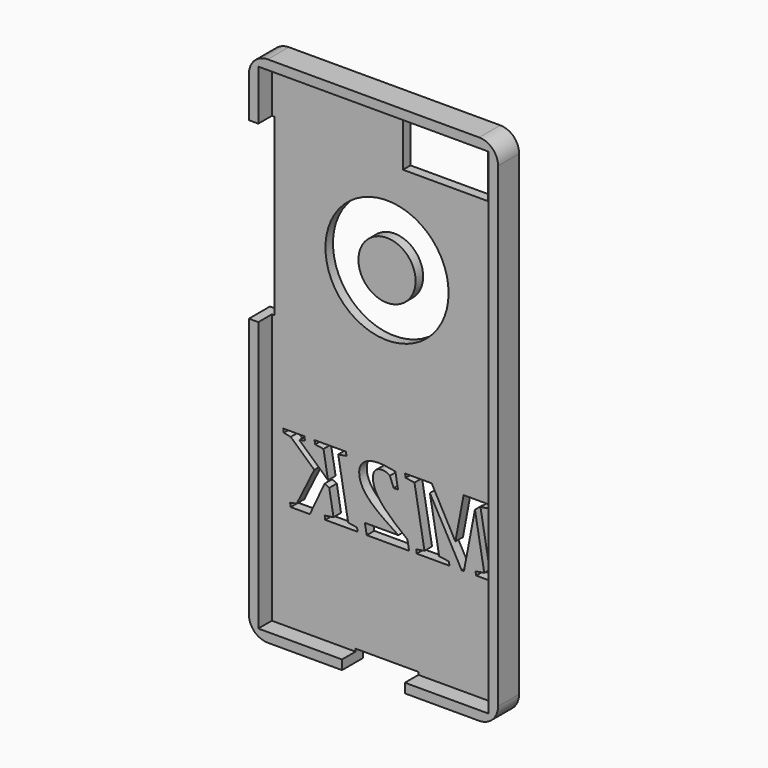
from build123d import *

# Parameters (mm, degrees)
F0_W          = 67.1
F0_H          = 138.3
F1_DEPTH      = 3.55
F2_T          = -2.54
F3_R          = 5.08
F4_W          = 22.9508173652
F4_H          = 12.0491795242
F5_DEPTH      = 12.5
F6_W          = 16.9322472066
F6_H          = 7.1
F7_DEPTH      = 3.25
F8_W          = 7.1
F8_H          = 47.0491815358
F9_DEPTH      = 3.25
F10_R         = 16.5823645395
F10_R_2       = 7.6979390502
F11_DEPTH     = 12.5
F12_TEXT_SIZE = 27.4609729899
F13_DEPTH     = 12.5


# Not quite as in the source:
# - Text() gives the source's letters only with a copy of the font that has no kerning and outlines rounded to 1/6400 em; it was checked with that copy


with BuildPart() as f1:
    # F0 (on Front) → F1 (new body, symmetric)
    with BuildSketch(Plane.XZ):
        Rectangle(F0_W, F0_H)
    extrude(amount=F1_DEPTH, both=True)

    # F2
    f2_openings = [f1.faces().sort_by_distance(p)[0] for p in [
        (0, -3.55, 0),
    ]]
    offset(amount=F2_T, openings=f2_openings)

    # F3
    f3_edges = [f1.edges().sort_by_distance(p)[0] for p in [
        (33.55, 0, 69.15),
        (33.55, 0, -69.15),
        (-33.55, 0, -69.15),
        (-33.55, 0, 69.15),
    ]]
    fillet(f3_edges, radius=F3_R)

    # F4 (on face) → F5 (cut, symmetric)
    with BuildSketch(Plane.XZ.offset(-1.01)):
        with Locations((15.7786884811, 57.8073803335)):
            Rectangle(F4_W, F4_H)
    extrude(amount=F5_DEPTH, both=True, mode=Mode.SUBTRACT)

    # F6 (on face) → F7 (cut, symmetric)
    with BuildSketch(Plane(origin=(0, 0, -69.15), x_dir=(1, 0, 0), z_dir=(0, 0, -1))):
        Rectangle(F6_W, F6_H)
    extrude(amount=F7_DEPTH, both=True, mode=Mode.SUBTRACT)

    # F8 (on face) → F9 (cut, symmetric)
    with BuildSketch(Plane(origin=(-33.55, 0, 0), x_dir=(0, -1, 0), z_dir=(-1, 0, 0))):
        with Locations((0, 29.54918053)):
            Rectangle(F8_W, F8_H)
    extrude(amount=F9_DEPTH, both=True, mode=Mode.SUBTRACT)

    # F10 (on face) → F11 (cut, symmetric)
    with BuildSketch(Plane.XZ.offset(-1.01)):
        with Locations((0, 26.536885649)):
            Circle(F10_R)
        with Locations((0, 26.536885649)):
            Circle(F10_R_2, mode=Mode.SUBTRACT)
    extrude(amount=F11_DEPTH, both=True, mode=Mode.SUBTRACT)

    # F12 (on face) → F13 (cut, symmetric)
    with BuildSketch(Plane(origin=(0, 3.55, 0), x_dir=(-1, 0, 0), z_dir=(0, 1, 0))):
        with Locations((-30.0354392077, -38.0229727307)):
            Text('M2K', F12_TEXT_SIZE, font='Tinos', font_style=FontStyle.BOLDITALIC, text_align=(TextAlign.LEFT, TextAlign.BOTTOM))
    extrude(amount=F13_DEPTH, both=True, mode=Mode.SUBTRACT)


solid = f1.part
